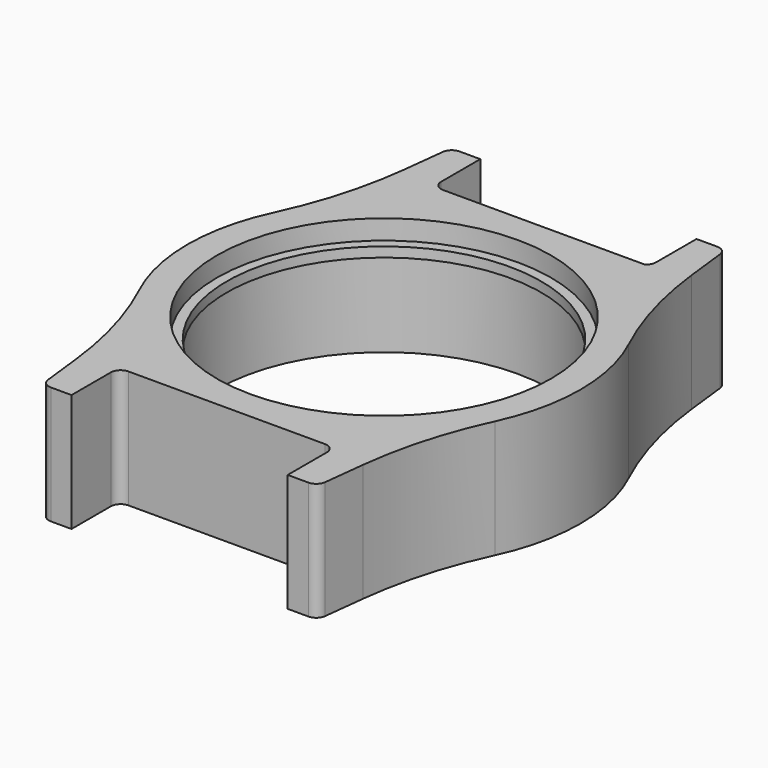
from build123d import *

# Parameters (mm, degrees)
F1_DEPTH = 12
F3_R     = 16
F4_DEPTH = 12.001
F5_R     = 17
F5_R_2   = 16
F6_DEPTH = 2
F2_R     = 17
F7_DEPTH = 9


# Not quite as in the source:
# - the program builds the solid bodies; features that only make, move or delete a surface that nothing else refers to are left out


with BuildPart() as f1:
    # F0 (on Top) → F1 (new body)
    with BuildSketch(Plane.XY):
        with BuildLine():
            Line((10.5367190596, 20), (0, 20))
            Line((0, 20), (-10, 20))
            ThreePointArc((-10, 20), (-10.7071067812, 20.2928932188), (-11, 21))
            Line((-11, 21), (-11, 26))
            Line((-11, 26), (-13.1087498209, 26))
            ThreePointArc((-13.1087498209, 26), (-13.7740978096, 25.7465333576), (-14.1021587568, 25.114624108))
            Line((-14.1021587568, 25.114624108), (-14.5904720191, 20.8825758343))
            ThreePointArc((-14.5904720191, 20.8825758343), (-15.8474732978, 14.5432941931), (-18.1089431513, 8.4891800512))
            ThreePointArc((-18.1089431513, 8.4891800512), (-20, 0), (-18.1089431513, -8.4891800512))
            ThreePointArc((-18.1089431513, -8.4891800512), (-15.8474732978, -14.5432941931), (-14.5904720191, -20.8825758343))
            Line((-14.5904720191, -20.8825758343), (-14.1021587568, -25.114624108))
            ThreePointArc((-14.1021587568, -25.114624108), (-13.7740978096, -25.7465333576), (-13.1087498209, -26))
            Line((-13.1087498209, -26), (-11, -26))
            Line((-11, -26), (-11, -21))
            ThreePointArc((-11, -21), (-10.7071067812, -20.2928932188), (-10, -20))
            Line((-10, -20), (0, -20))
            Line((0, -20), (10, -20))
            ThreePointArc((10, -20), (10.7071067812, -20.2928932188), (11, -21))
            Line((11, -21), (11, -26))
            Line((11, -26), (13.1087498209, -26))
            ThreePointArc((13.1087498209, -26), (13.7740978096, -25.7465333576), (14.1021587568, -25.114624108))
            Line((14.1021587568, -25.114624108), (14.5904720191, -20.8825758343))
            ThreePointArc((14.5904720191, -20.8825758343), (15.8474732978, -14.5432941931), (18.1089431513, -8.4891800512))
            ThreePointArc((18.1089431513, -8.4891800512), (20, 0), (18.1089431513, 8.4891800512))
            ThreePointArc((18.1089431513, 8.4891800512), (15.8474732978, 14.5432941931), (14.5904720191, 20.8825758343))
            Line((14.5904720191, 20.8825758343), (14.1021587568, 25.114624108))
            ThreePointArc((14.1021587568, 25.114624108), (13.7740978096, 25.7465333576), (13.1087498209, 26))
            Line((13.1087498209, 26), (11, 26))
            Line((11, 26), (11, 20.8437610154))
            ThreePointArc((11, 20.8437610154), (10.8765611957, 20.3624705935), (10.5367190596, 20))
        make_face()
    extrude(amount=F1_DEPTH)

    # F3 (on face) → F4 (cut, through all)
    with BuildSketch(Plane.XY.offset(12)):
        Circle(F3_R)
    extrude(amount=-F4_DEPTH, mode=Mode.SUBTRACT)

    # F5 (on face) → F6 (cut)
    with BuildSketch(Plane.XY.offset(12)):
        Circle(F5_R)
        Circle(F5_R_2, mode=Mode.SUBTRACT)
    extrude(amount=-F6_DEPTH, mode=Mode.SUBTRACT)

    # F2 (on face) → F7 (cut)
    with BuildSketch(Plane(origin=(0, 0, 0), x_dir=(1, 0, 0), z_dir=(0, 0, -1))):
        Circle(F2_R)
    extrude(amount=-F7_DEPTH, mode=Mode.SUBTRACT)


solid = f1.part
